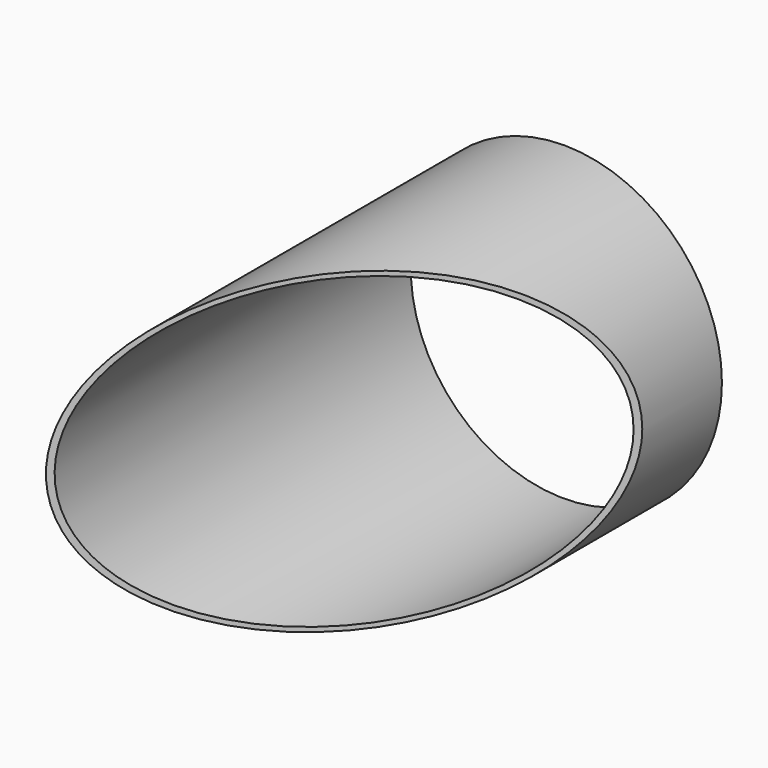
from build123d import *

# Parameters (mm, degrees)
F0_R        = 51.5
F0_R_2      = 50
F1_DEPTH    = 160
F1_FACE_R   = 51.5
F1_FACE_R_2 = 50
F4_REACH    = 273.1919484463


with BuildPart() as f1:
    # F0 (on Front) → F1 (new body)
    with BuildSketch(Plane.XZ):
        Circle(F0_R)
        Circle(F0_R_2, mode=Mode.SUBTRACT)
    extrude(amount=F1_DEPTH)

    f4_end = Plane(origin=(44.5886895286, -40.1478363815, 0), x_dir=(0.6691306064, 0.7431448255, 0), z_dir=(0.7431448255, -0.6691306064, 0))
    # F1_face (on face) → F4 (cut, up to a plane its end follows)
    with BuildSketch(Plane.XZ.offset(160)):
        Circle(F1_FACE_R)
        Circle(F1_FACE_R_2, mode=Mode.SUBTRACT)
    f4_long = extrude(amount=-F4_REACH, mode=Mode.PRIVATE)
    add(split(f4_long, bisect_by=f4_end, keep=Keep.TOP, mode=Mode.PRIVATE), mode=Mode.SUBTRACT)


solid = f1.part
